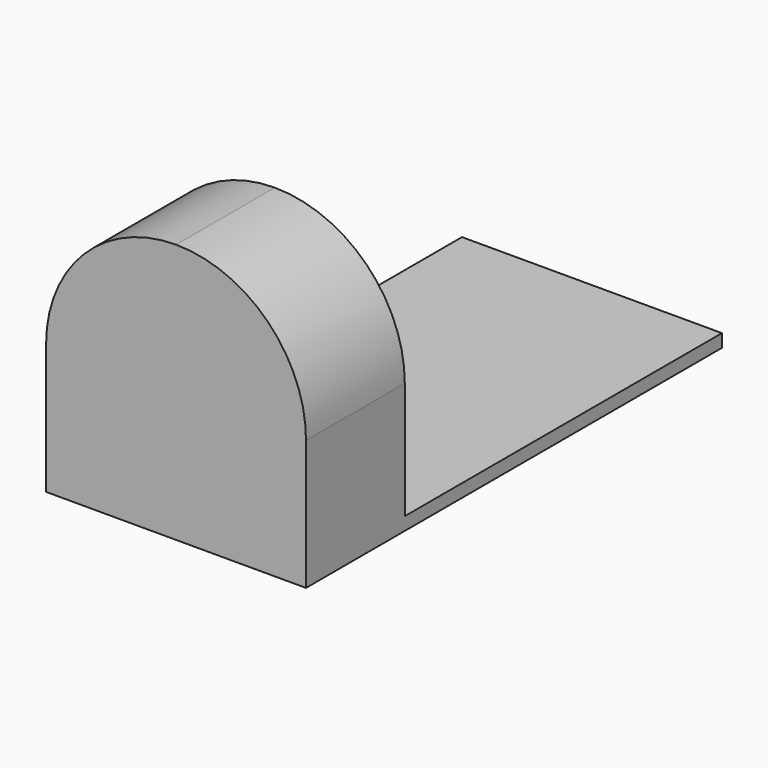
from build123d import *

# Parameters (mm, degrees)
F0_W     = 40
F0_H     = 61
F1_DEPTH = 2
F0_H_2   = 19
F2_DEPTH = 40
F3_R     = 18
F4_DEPTH = 17
F5_R     = 19.99999


# Not quite as in the source:
# - a fillet or chamfer is up to 0.001 mm smaller than in the source, because OpenCascade refuses the exact size


with BuildPart() as f1:
    # F0 (on Top) → F1 (new body)
    with BuildSketch(Plane.XY):
        with Locations((-2.8480109572, 28.6193176061)):
            Rectangle(F0_W, F0_H)
    extrude(amount=F1_DEPTH)

    # F0 (on Top) → F2 (join)
    with BuildSketch(Plane.XY):
        with Locations((-2.8480109572, -11.3806823939)):
            Rectangle(F0_W, F0_H_2)
    extrude(amount=F2_DEPTH)

    # F3 (on face) → F4 (cut)
    with BuildSketch(Plane(origin=(0, -1.8806823939, 0), x_dir=(-1, 0, 0), z_dir=(0, 1, 0))):
        with Locations((2.8480109572, 21)):
            Circle(F3_R)
    extrude(amount=-F4_DEPTH, mode=Mode.SUBTRACT)

    # F5 (radius 20 in the source; OpenCascade refuses exactly that, so slightly less here)
    f5_edges = [f1.edges().sort_by_distance(p)[0] for p in [
        (17.151989, -11.380682, 40),
        (-22.848011, -11.380682, 40),
    ]]
    fillet(f5_edges, radius=F5_R)


solid = f1.part
